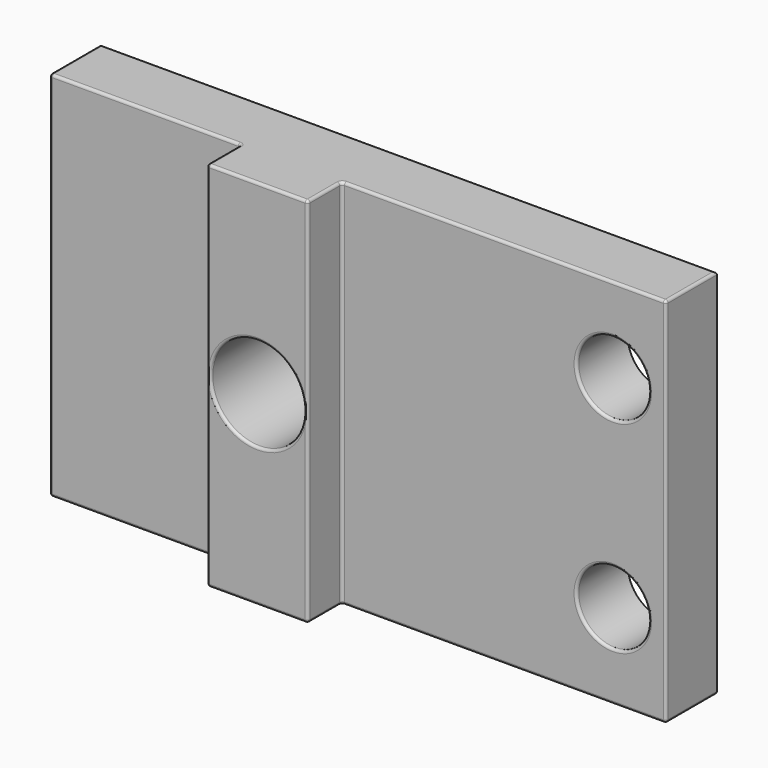
from build123d import *

# Parameters (mm, degrees)
F0_W         = 58
F0_H         = 35
F1_DEPTH     = 6
F2_W         = 9.5
F2_H         = 35
F3_DEPTH     = 4
F4_D         = 6.8
F6_D         = 8.8
F7_T1_DEPTH  = 35
F7_T3_DEPTH  = 36.25
F7_T5_DEPTH  = 10.75
F7_T7_DEPTH  = 7.25
F7_T9_DEPTH  = 6.375
F7_T11_DEPTH = 58.375
F7_T13_DEPTH = 34.5
F7_S17_W     = 0.25
F7_S17_H     = 0.25
F7_T18_DEPTH = 0.25
F7_S23_W     = 0.25
F7_S23_H     = 0.25
F7_T24_DEPTH = 0.25
F7_T33_DEPTH = 30
F7_T35_DEPTH = 17.5
F7_T37_DEPTH = 3.5
F7_S41_W     = 0.25
F7_S41_H     = 0.25
F7_T42_DEPTH = 0.25
F7_S47_W     = 0.25
F7_S47_H     = 0.25
F7_T48_DEPTH = 0.25
F7_S53_W     = 0.25
F7_S53_H     = 0.25
F7_T54_DEPTH = 0.25
F7_S59_W     = 0.25
F7_S59_H     = 0.25
F7_T60_DEPTH = 0.25
F7_S65_W     = 0.25
F7_S65_H     = 0.25
F7_T66_DEPTH = 0.25
F7_S71_W     = 0.25
F7_S71_H     = 0.25
F7_T72_DEPTH = 0.25
F7_S77_W     = 0.25
F7_S77_H     = 0.25
F7_T78_DEPTH = 0.25
F7_S83_W     = 0.25
F7_S83_H     = 0.25
F7_T84_DEPTH = 0.25
F7_T88_ANGLE = 90
F7_T90_ANGLE = 90
F7_T92_ANGLE = 90
F7_T94_ANGLE = 90


# Not quite as in the source:
# - a fillet or chamfer that OpenCascade refuses, or shapes differently, is made with other operations: its cross-section is extruded or revolved along the edge and cut away or added


with BuildPart() as f1:
    # F0 (on Front) → F1 (new body)
    with BuildSketch(Plane.XZ):
        Rectangle(F0_W, F0_H)
    extrude(amount=F1_DEPTH)

    # F2 (on face) → F3 (join)
    with BuildSketch(Plane.XZ.offset(6)):
        with Locations((-6.25, 0)):
            Rectangle(F2_W, F2_H)
    extrude(amount=F3_DEPTH)

    # F4 (through all)
    with Locations(Plane.XZ.offset(6)):
        with Locations((24, 9.5), (24, -9.5)):
            Hole(F4_D / 2)

    # F6 (through all)
    with Locations(Plane.XZ.offset(10)):
        with Locations((-6.25, 0)):
            Hole(F6_D / 2)

    # F7: fillet of radius 0.25 on 26 edges, made by hand

    # F7_s2 → F7_t1 (join)
    with BuildSketch(Plane.XY.offset(-17.5)):
        with BuildLine():
            ThreePointArc((-1.25, -6), (-1.4267766953, -6.0732233047), (-1.5, -6.25))
            Line((-1.5, -6.25), (-1.5, -6))
            Line((-1.5, -6), (-1.25, -6))
        make_face()
        with BuildLine():
            ThreePointArc((-11.25, -6), (-11.0732233047, -6.0732233047), (-11, -6.25))
            Line((-11, -6.25), (-11, -6))
            Line((-11, -6), (-11.25, -6))
        make_face()
    extrude(amount=F7_T1_DEPTH)

    # F7_s4 → F7_t3 (cut)
    with BuildSketch(Plane.XY.offset(-18.125)):
        with BuildLine():
            ThreePointArc((29, -5.75), (28.9267766953, -5.9267766953), (28.75, -6))
            Line((28.75, -6), (29, -6))
            Line((29, -6), (29, -5.75))
        make_face()
        with BuildLine():
            ThreePointArc((-11, -9.75), (-10.9267766953, -9.9267766953), (-10.75, -10))
            Line((-10.75, -10), (-11, -10))
            Line((-11, -10), (-11, -9.75))
        make_face()
        with BuildLine():
            ThreePointArc((-1.75, -10), (-1.5732233047, -9.9267766953), (-1.5, -9.75))
            Line((-1.5, -9.75), (-1.5, -10))
            Line((-1.5, -10), (-1.75, -10))
        make_face()
        with BuildLine():
            ThreePointArc((-29, -5.75), (-28.9267766953, -5.9267766953), (-28.75, -6))
            Line((-28.75, -6), (-29, -6))
            Line((-29, -6), (-29, -5.75))
        make_face()
    extrude(amount=F7_T3_DEPTH, mode=Mode.SUBTRACT)

    # F7_s6 → F7_t5 (cut)
    with BuildSketch(Plane.YZ.offset(-11.625)):
        with BuildLine():
            ThreePointArc((-9.75, 17.5), (-9.9267766953, 17.4267766953), (-10, 17.25))
            Line((-10, 17.25), (-10, 17.5))
            Line((-10, 17.5), (-9.75, 17.5))
        make_face()
        with BuildLine():
            ThreePointArc((-9.75, -17.5), (-9.9267766953, -17.4267766953), (-10, -17.25))
            Line((-10, -17.25), (-10, -17.5))
            Line((-10, -17.5), (-9.75, -17.5))
        make_face()
    extrude(amount=F7_T5_DEPTH, mode=Mode.SUBTRACT)

    # F7_s8 → F7_t7 (cut)
    with BuildSketch(Plane.XZ.offset(-0.625)):
        with BuildLine():
            ThreePointArc((29, 17.25), (28.9267766953, 17.4267766953), (28.75, 17.5))
            Line((28.75, 17.5), (29, 17.5))
            Line((29, 17.5), (29, 17.25))
        make_face()
        with BuildLine():
            ThreePointArc((29, -17.25), (28.9267766953, -17.4267766953), (28.75, -17.5))
            Line((28.75, -17.5), (29, -17.5))
            Line((29, -17.5), (29, -17.25))
        make_face()
    extrude(amount=F7_T7_DEPTH, mode=Mode.SUBTRACT)

    # F7_s10 → F7_t9 (cut)
    with BuildSketch(Plane.XZ.offset(0.25)):
        with BuildLine():
            ThreePointArc((-28.75, 17.5), (-28.9267766953, 17.4267766953), (-29, 17.25))
            Line((-29, 17.25), (-29, 17.5))
            Line((-29, 17.5), (-28.75, 17.5))
        make_face()
        with BuildLine():
            ThreePointArc((-28.75, -17.5), (-28.9267766953, -17.4267766953), (-29, -17.25))
            Line((-29, -17.25), (-29, -17.5))
            Line((-29, -17.5), (-28.75, -17.5))
        make_face()
    extrude(amount=F7_T9_DEPTH, mode=Mode.SUBTRACT)

    # F7_s12 → F7_t11 (cut)
    with BuildSketch(Plane.YZ.offset(-28.75)):
        with BuildLine():
            ThreePointArc((-0.25, 17.5), (-0.0732233047, 17.4267766953), (0, 17.25))
            Line((0, 17.25), (0, 17.5))
            Line((0, 17.5), (-0.25, 17.5))
        make_face()
        with BuildLine():
            ThreePointArc((-0.25, -17.5), (-0.0732233047, -17.4267766953), (0, -17.25))
            Line((0, -17.25), (0, -17.5))
            Line((0, -17.5), (-0.25, -17.5))
        make_face()
    extrude(amount=F7_T11_DEPTH, mode=Mode.SUBTRACT)

    # F7_s14 → F7_t13 (cut)
    with BuildSketch(Plane.XY.offset(-17.25)):
        with BuildLine():
            ThreePointArc((-28.75, 0), (-28.9267766953, -0.0732233047), (-29, -0.25))
            Line((-29, -0.25), (-29, 0))
            Line((-29, 0), (-28.75, 0))
        make_face()
    extrude(amount=F7_T13_DEPTH, mode=Mode.SUBTRACT)


with BuildPart() as f7_tool16:
    # F7_s17 → F7_t18 (new body)
    with BuildSketch(Plane.XY.offset(17.25)):
        with Locations((-28.875, -0.125)):
            Rectangle(F7_S17_W, F7_S17_H)
    extrude(amount=F7_T18_DEPTH)

    # F7_s19 → F7_t20 (revolve, cut)
    with BuildSketch(Plane(origin=(-28.75, -0.25, 17.25), x_dir=(0.7071067812, -0.7071067812, 0), z_dir=(-0.7071067812, -0.7071067812, 0))):
        with BuildLine():
            ThreePointArc((0, -0.25), (0.25, 0), (0, 0.25))
            Line((0, 0.25), (0, -0.25))
        make_face()
    revolve(axis=Axis((-28.75, -0.25, 17.25), (0, 0, 1)), mode=Mode.SUBTRACT)


with BuildPart() as f1_1:
    add(f1.part)

    # F7_t15: cut F7_tool16
    add(f7_tool16.part, mode=Mode.SUBTRACT)


with BuildPart() as f7_tool22:
    # F7_s23 → F7_t24 (new body)
    with BuildSketch(Plane.XY.offset(-17.25)):
        with Locations((-28.875, -0.125)):
            Rectangle(F7_S23_W, F7_S23_H)
    extrude(amount=-F7_T24_DEPTH)

    # F7_s25 → F7_t26 (revolve, cut)
    with BuildSketch(Plane(origin=(-28.75, -0.25, -17.25), x_dir=(0.7071067812, -0.7071067812, 0), z_dir=(0.7071067812, 0.7071067812, 0))):
        with BuildLine():
            ThreePointArc((0, -0.25), (0.25, 0), (0, 0.25))
            Line((0, 0.25), (0, -0.25))
        make_face()
    revolve(axis=Axis((-28.75, -0.25, -17.25), (0, 0, -1)), mode=Mode.SUBTRACT)


with BuildPart() as f1_2:
    add(f1_1.part)

    # F7_t21: cut F7_tool22
    add(f7_tool22.part, mode=Mode.SUBTRACT)

    # F7_s27 → F7_t28 (revolve, cut)
    with BuildSketch(Plane.XY.offset(-9.5)):
        with BuildLine():
            ThreePointArc((27.65, -6), (27.4732233047, -5.9267766953), (27.4, -5.75))
            Line((27.4, -5.75), (27.4, -6))
            Line((27.4, -6), (27.65, -6))
        make_face()
    revolve(axis=Axis((24, -6, -9.5), (0, -1, 0)), mode=Mode.SUBTRACT)

    # F7_s29 → F7_t30 (revolve, cut)
    with BuildSketch(Plane.XY.offset(9.5)):
        with BuildLine():
            ThreePointArc((27.65, -6), (27.4732233047, -5.9267766953), (27.4, -5.75))
            Line((27.4, -5.75), (27.4, -6))
            Line((27.4, -6), (27.65, -6))
        make_face()
    revolve(axis=Axis((24, -6, 9.5), (0, -1, 0)), mode=Mode.SUBTRACT)

    # F7_s31 → F7_t32 (revolve, cut)
    with BuildSketch(Plane.XY):
        with BuildLine():
            ThreePointArc((-1.6, -10), (-1.7767766953, -9.9267766953), (-1.85, -9.75))
            Line((-1.85, -9.75), (-1.85, -10))
            Line((-1.85, -10), (-1.6, -10))
        make_face()
    revolve(axis=Axis((-6.25, -10, 0), (0, -1, 0)), mode=Mode.SUBTRACT)

    # F7_s34 → F7_t33 (cut)
    with BuildSketch(Plane.YZ.offset(-1.25)):
        with BuildLine():
            ThreePointArc((-6, -17.25), (-5.9267766953, -17.4267766953), (-5.75, -17.5))
            Line((-5.75, -17.5), (-6, -17.5))
            Line((-6, -17.5), (-6, -17.25))
        make_face()
        with BuildLine():
            ThreePointArc((-5.75, 17.5), (-5.9267766953, 17.4267766953), (-6, 17.25))
            Line((-6, 17.25), (-6, 17.5))
            Line((-6, 17.5), (-5.75, 17.5))
        make_face()
    extrude(amount=F7_T33_DEPTH, mode=Mode.SUBTRACT)

    # F7_s36 → F7_t35 (cut)
    with BuildSketch(Plane.YZ.offset(-28.75)):
        with BuildLine():
            ThreePointArc((-5.75, -17.5), (-5.9267766953, -17.4267766953), (-6, -17.25))
            Line((-6, -17.25), (-6, -17.5))
            Line((-6, -17.5), (-5.75, -17.5))
        make_face()
        with BuildLine():
            ThreePointArc((-5.75, 17.5), (-5.9267766953, 17.4267766953), (-6, 17.25))
            Line((-6, 17.25), (-6, 17.5))
            Line((-6, 17.5), (-5.75, 17.5))
        make_face()
    extrude(amount=F7_T35_DEPTH, mode=Mode.SUBTRACT)

    # F7_s38 → F7_t37 (cut)
    with BuildSketch(Plane.XZ.offset(6.25)):
        with BuildLine():
            ThreePointArc((-1.75, 17.5), (-1.5732233047, 17.4267766953), (-1.5, 17.25))
            Line((-1.5, 17.25), (-1.5, 17.5))
            Line((-1.5, 17.5), (-1.75, 17.5))
        make_face()
        with BuildLine():
            ThreePointArc((-10.75, 17.5), (-10.9267766953, 17.4267766953), (-11, 17.25))
            Line((-11, 17.25), (-11, 17.5))
            Line((-11, 17.5), (-10.75, 17.5))
        make_face()
        with BuildLine():
            ThreePointArc((-10.75, -17.5), (-10.9267766953, -17.4267766953), (-11, -17.25))
            Line((-11, -17.25), (-11, -17.5))
            Line((-11, -17.5), (-10.75, -17.5))
        make_face()
        with BuildLine():
            ThreePointArc((-1.75, -17.5), (-1.5732233047, -17.4267766953), (-1.5, -17.25))
            Line((-1.5, -17.25), (-1.5, -17.5))
            Line((-1.5, -17.5), (-1.75, -17.5))
        make_face()
    extrude(amount=F7_T37_DEPTH, mode=Mode.SUBTRACT)


with BuildPart() as f7_tool40:
    # F7_s41 → F7_t42 (new body)
    with BuildSketch(Plane.XY.offset(-17.25)):
        with Locations((-1.625, -9.875)):
            Rectangle(F7_S41_W, F7_S41_H)
    extrude(amount=-F7_T42_DEPTH)

    # F7_s43 → F7_t44 (revolve, cut)
    with BuildSketch(Plane(origin=(-1.75, -9.75, -17.25), x_dir=(-0.7071067812, 0.7071067812, 0), z_dir=(-0.7071067812, -0.7071067812, 0))):
        with BuildLine():
            ThreePointArc((0, -0.25), (0.25, 0), (0, 0.25))
            Line((0, 0.25), (0, -0.25))
        make_face()
    revolve(axis=Axis((-1.75, -9.75, -17.25), (0, 0, -1)), mode=Mode.SUBTRACT)


with BuildPart() as f1_3:
    add(f1_2.part)

    # F7_t39: cut F7_tool40
    add(f7_tool40.part, mode=Mode.SUBTRACT)


with BuildPart() as f7_tool46:
    # F7_s47 → F7_t48 (new body)
    with BuildSketch(Plane.XY.offset(-17.25)):
        with Locations((-10.875, -9.875)):
            Rectangle(F7_S47_W, F7_S47_H)
    extrude(amount=-F7_T48_DEPTH)

    # F7_s49 → F7_t50 (revolve, cut)
    with BuildSketch(Plane(origin=(-10.75, -9.75, -17.25), x_dir=(0.7071067812, 0.7071067812, 0), z_dir=(-0.7071067812, 0.7071067812, 0))):
        with BuildLine():
            ThreePointArc((0, -0.25), (0.25, 0), (0, 0.25))
            Line((0, 0.25), (0, -0.25))
        make_face()
    revolve(axis=Axis((-10.75, -9.75, -17.25), (0, 0, -1)), mode=Mode.SUBTRACT)


with BuildPart() as f1_4:
    add(f1_3.part)

    # F7_t45: cut F7_tool46
    add(f7_tool46.part, mode=Mode.SUBTRACT)


with BuildPart() as f7_tool52:
    # F7_s53 → F7_t54 (new body)
    with BuildSketch(Plane.XY.offset(17.25)):
        with Locations((-10.875, -9.875)):
            Rectangle(F7_S53_W, F7_S53_H)
    extrude(amount=F7_T54_DEPTH)

    # F7_s55 → F7_t56 (revolve, cut)
    with BuildSketch(Plane(origin=(-10.75, -9.75, 17.25), x_dir=(0.7071067812, 0.7071067812, 0), z_dir=(0.7071067812, -0.7071067812, 0))):
        with BuildLine():
            ThreePointArc((0, -0.25), (0.25, 0), (0, 0.25))
            Line((0, 0.25), (0, -0.25))
        make_face()
    revolve(axis=Axis((-10.75, -9.75, 17.25), (0, 0, 1)), mode=Mode.SUBTRACT)


with BuildPart() as f1_5:
    add(f1_4.part)

    # F7_t51: cut F7_tool52
    add(f7_tool52.part, mode=Mode.SUBTRACT)


with BuildPart() as f7_tool58:
    # F7_s59 → F7_t60 (new body)
    with BuildSketch(Plane.XY.offset(17.25)):
        with Locations((-1.625, -9.875)):
            Rectangle(F7_S59_W, F7_S59_H)
    extrude(amount=F7_T60_DEPTH)

    # F7_s61 → F7_t62 (revolve, cut)
    with BuildSketch(Plane(origin=(-1.75, -9.75, 17.25), x_dir=(-0.7071067812, 0.7071067812, 0), z_dir=(0.7071067812, 0.7071067812, 0))):
        with BuildLine():
            ThreePointArc((0, -0.25), (0.25, 0), (0, 0.25))
            Line((0, 0.25), (0, -0.25))
        make_face()
    revolve(axis=Axis((-1.75, -9.75, 17.25), (0, 0, 1)), mode=Mode.SUBTRACT)


with BuildPart() as f1_6:
    add(f1_5.part)

    # F7_t57: cut F7_tool58
    add(f7_tool58.part, mode=Mode.SUBTRACT)


with BuildPart() as f7_tool64:
    # F7_s65 → F7_t66 (new body)
    with BuildSketch(Plane.XY.offset(17.25)):
        with Locations((-28.875, -5.875)):
            Rectangle(F7_S65_W, F7_S65_H)
    extrude(amount=F7_T66_DEPTH)

    # F7_s67 → F7_t68 (revolve, cut)
    with BuildSketch(Plane(origin=(-28.75, -5.75, 17.25), x_dir=(0.7071067812, 0.7071067812, 0), z_dir=(0.7071067812, -0.7071067812, 0))):
        with BuildLine():
            ThreePointArc((0, -0.25), (0.25, 0), (0, 0.25))
            Line((0, 0.25), (0, -0.25))
        make_face()
    revolve(axis=Axis((-28.75, -5.75, 17.25), (0, 0, 1)), mode=Mode.SUBTRACT)


with BuildPart() as f1_7:
    add(f1_6.part)

    # F7_t63: cut F7_tool64
    add(f7_tool64.part, mode=Mode.SUBTRACT)


with BuildPart() as f7_tool70:
    # F7_s71 → F7_t72 (new body)
    with BuildSketch(Plane.XY.offset(-17.25)):
        with Locations((-28.875, -5.875)):
            Rectangle(F7_S71_W, F7_S71_H)
    extrude(amount=-F7_T72_DEPTH)

    # F7_s73 → F7_t74 (revolve, cut)
    with BuildSketch(Plane(origin=(-28.75, -5.75, -17.25), x_dir=(0.7071067812, 0.7071067812, 0), z_dir=(-0.7071067812, 0.7071067812, 0))):
        with BuildLine():
            ThreePointArc((0, -0.25), (0.25, 0), (0, 0.25))
            Line((0, 0.25), (0, -0.25))
        make_face()
    revolve(axis=Axis((-28.75, -5.75, -17.25), (0, 0, -1)), mode=Mode.SUBTRACT)


with BuildPart() as f1_8:
    add(f1_7.part)

    # F7_t69: cut F7_tool70
    add(f7_tool70.part, mode=Mode.SUBTRACT)


with BuildPart() as f7_tool76:
    # F7_s77 → F7_t78 (new body)
    with BuildSketch(Plane.XY.offset(17.25)):
        with Locations((28.875, -5.875)):
            Rectangle(F7_S77_W, F7_S77_H)
    extrude(amount=F7_T78_DEPTH)

    # F7_s79 → F7_t80 (revolve, cut)
    with BuildSketch(Plane(origin=(28.75, -5.75, 17.25), x_dir=(-0.7071067812, 0.7071067812, 0), z_dir=(0.7071067812, 0.7071067812, 0))):
        with BuildLine():
            ThreePointArc((0, -0.25), (0.25, 0), (0, 0.25))
            Line((0, 0.25), (0, -0.25))
        make_face()
    revolve(axis=Axis((28.75, -5.75, 17.25), (0, 0, 1)), mode=Mode.SUBTRACT)


with BuildPart() as f1_9:
    add(f1_8.part)

    # F7_t75: cut F7_tool76
    add(f7_tool76.part, mode=Mode.SUBTRACT)


with BuildPart() as f7_tool82:
    # F7_s83 → F7_t84 (new body)
    with BuildSketch(Plane.XZ.offset(5.75)):
        with Locations((28.875, -17.375)):
            Rectangle(F7_S83_W, F7_S83_H)
    extrude(amount=F7_T84_DEPTH)

    # F7_s85 → F7_t86 (revolve, cut)
    with BuildSketch(Plane(origin=(28.75, -5.75, -17.25), x_dir=(-0.7071067812, 0, 0.7071067812), z_dir=(0.7071067812, 0, 0.7071067812))):
        with BuildLine():
            ThreePointArc((0, -0.25), (0.25, 0), (0, 0.25))
            Line((0, 0.25), (0, -0.25))
        make_face()
    revolve(axis=Axis((28.75, -5.75, -17.25), (0, -1, 0)), mode=Mode.SUBTRACT)


with BuildPart() as f1_10:
    add(f1_9.part)

    # F7_t81: cut F7_tool82
    add(f7_tool82.part, mode=Mode.SUBTRACT)

    # F7_s87 → F7_t88 (revolve, cut)
    with BuildSketch(Plane.YZ.offset(-1.25)):
        with BuildLine():
            ThreePointArc((-5.75, -17.5), (-5.9267766953, -17.4267766953), (-6, -17.25))
            Line((-6, -17.25), (-6, -17.5))
            Line((-6, -17.5), (-5.75, -17.5))
        make_face()
    revolve(axis=Axis((-1.25, -6.25, -17.5), (0, 0, 1)), revolution_arc=F7_T88_ANGLE, mode=Mode.SUBTRACT)

    # F7_s89 → F7_t90 (revolve, cut)
    with BuildSketch(Plane.YZ.offset(-11.25)):
        with BuildLine():
            ThreePointArc((-5.75, -17.5), (-5.9267766953, -17.4267766953), (-6, -17.25))
            Line((-6, -17.25), (-6, -17.5))
            Line((-6, -17.5), (-5.75, -17.5))
        make_face()
    revolve(axis=Axis((-11.25, -6.25, -17.5), (0, 0, -1)), revolution_arc=F7_T90_ANGLE, mode=Mode.SUBTRACT)

    # F7_s91 → F7_t92 (revolve, cut)
    with BuildSketch(Plane.YZ.offset(-11.25)):
        with BuildLine():
            ThreePointArc((-5.75, 17.5), (-5.9267766953, 17.4267766953), (-6, 17.25))
            Line((-6, 17.25), (-6, 17.5))
            Line((-6, 17.5), (-5.75, 17.5))
        make_face()
    revolve(axis=Axis((-11.25, -6.25, 17.5), (0, 0, -1)), revolution_arc=F7_T92_ANGLE, mode=Mode.SUBTRACT)

    # F7_s93 → F7_t94 (revolve, cut)
    with BuildSketch(Plane.YZ.offset(-1.25)):
        with BuildLine():
            ThreePointArc((-5.75, 17.5), (-5.9267766953, 17.4267766953), (-6, 17.25))
            Line((-6, 17.25), (-6, 17.5))
            Line((-6, 17.5), (-5.75, 17.5))
        make_face()
    revolve(axis=Axis((-1.25, -6.25, 17.5), (0, 0, 1)), revolution_arc=F7_T94_ANGLE, mode=Mode.SUBTRACT)


solid = f1_10.part
